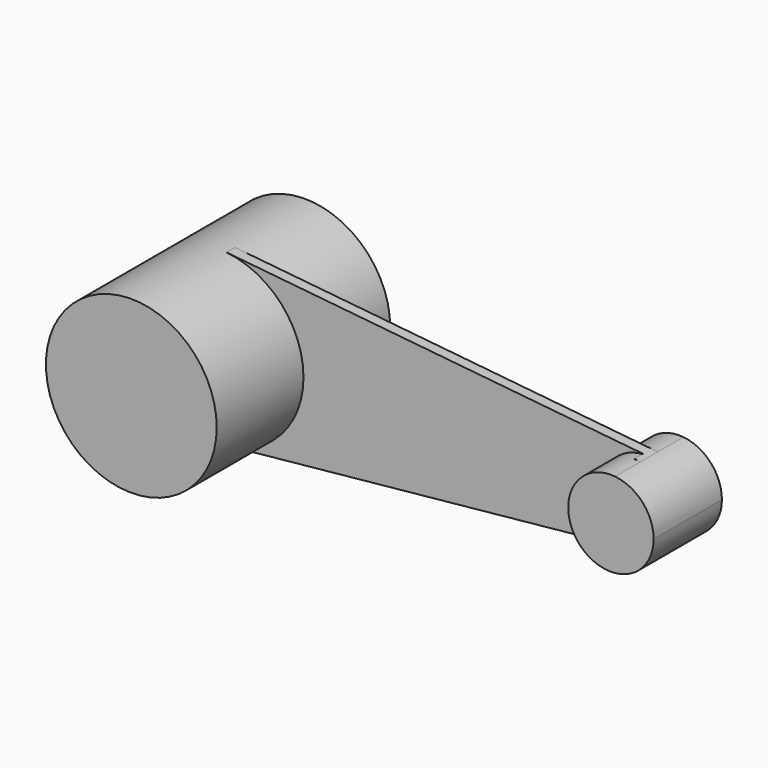
from build123d import *

# Parameters (mm, degrees)
F1_DEPTH   = 2.5
F2_DEPTH   = 5
F3_DEPTH   = 1.25
F5_D       = 100
F5_DEPTH   = 12.7
F5_TIP     = 30.0430309514
F5_2_D     = 100
F5_2_DEPTH = 12.7
F5_2_TIP   = 30.0430309514
F6_DEPTH   = 12.7


# Not quite as in the source:
# - a feature of the source that left no trace in its solid (it failed there, or was rolled back) is left out


with BuildPart() as f1:
    # F0 (on Front) → F1 (new body, symmetric)
    with BuildSketch(Plane.XZ):
        with BuildLine():
            ThreePointArc((-40, 0), (-42.5838015129, 6.7082039325), (-49, 9.9498743711))
            ThreePointArc((-49, 9.9498743711), (-60, 0), (-49, -9.9498743711))
            ThreePointArc((-49, -9.9498743711), (-42.5838015129, -6.7082039325), (-40, 0))
        make_face()
    extrude(amount=F1_DEPTH, both=True)

    # F5 (one way)
    with BuildSketch(Plane(origin=(0, 0, 0), x_dir=(1, 0, 0), z_dir=(0, 1, 0))):
        with Locations((-50, 0)):
            Circle(F5_D / 2)
    extrude(amount=-F5_DEPTH, mode=Mode.SUBTRACT)
    with Locations(Plane(origin=(0, 0, 0), x_dir=(1, 0, 0), z_dir=(0, 1, 0))):
        with Locations((-50, 0)):
            with Locations((0, 0, -(F5_DEPTH + F5_TIP / 2))):  # 118° drill point
                Cone(0, F5_D / 2, F5_TIP, mode=Mode.SUBTRACT)



with BuildPart() as f2:
    # F0 (on Front) → F2 (new body, symmetric)
    with BuildSketch(Plane.XZ):
        with BuildLine():
            ThreePointArc((0.5, -4.9749371855), (3.7080992435, -3.3541019662), (5, 0))
            ThreePointArc((5, 0), (3.7080992435, 3.3541019662), (0.5, 4.9749371855))
            ThreePointArc((0.5, 4.9749371855), (-5, 0), (0.5, -4.9749371855))
        make_face()
    extrude(amount=F2_DEPTH, both=True)


with BuildPart() as f3:
    # F0 (on Front) → F3 (new body, symmetric)
    with BuildSketch(Plane.XZ):
        with BuildLine():
            ThreePointArc((0.5, -4.9749371855), (-5, 0), (0.5, 4.9749371855))
            Line((0.5, 4.9749371855), (-49, 9.9498743711))
            ThreePointArc((-49, 9.9498743711), (-42.5838015129, 6.7082039325), (-40, 0))
            ThreePointArc((-40, 0), (-42.5838015129, -6.7082039325), (-49, -9.9498743711))
            Line((-49, -9.9498743711), (0.5, -4.9749371855))
        make_face()
    extrude(amount=F3_DEPTH, both=True)

    # F5#2 (one way)
    with BuildSketch(Plane(origin=(0, 0, 0), x_dir=(1, 0, 0), z_dir=(0, 1, 0))):
        with Locations((-50, 0)):
            Circle(F5_2_D / 2)
    extrude(amount=-F5_2_DEPTH, mode=Mode.SUBTRACT)
    with Locations(Plane(origin=(0, 0, 0), x_dir=(1, 0, 0), z_dir=(0, 1, 0))):
        with Locations((-50, 0)):
            with Locations((0, 0, -(F5_2_DEPTH + F5_2_TIP / 2))):  # 118° drill point
                Cone(0, F5_2_D / 2, F5_2_TIP, mode=Mode.SUBTRACT)


with BuildPart() as f1_1:
    add(f1.part)

    add(f3.part)  # F6 merges F3
    # F0 (on Front) → F6 (join, symmetric)
    with BuildSketch(Plane.XZ):
        with BuildLine():
            ThreePointArc((-40, 0), (-42.5838015129, 6.7082039325), (-49, 9.9498743711))
            ThreePointArc((-49, 9.9498743711), (-60, 0), (-49, -9.9498743711))
            ThreePointArc((-49, -9.9498743711), (-42.5838015129, -6.7082039325), (-40, 0))
        make_face()
    extrude(amount=F6_DEPTH, both=True)


solid = Compound([f2.part, f1_1.part])
